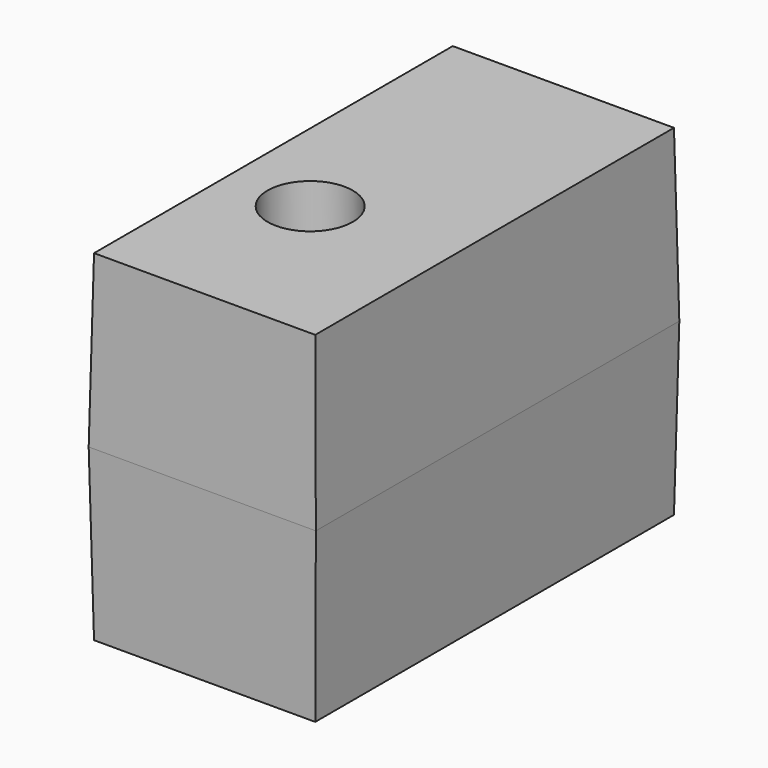
from build123d import *

# Parameters (mm, degrees)
F0_W           = 40
F0_H           = 80
F1_DEPTH       = 30
F1_TAPER       = 1
F3_D           = 9
F3_CBORE_D     = 15
F3_CBORE_DEPTH = 10


with BuildPart() as f1:
    # F0 (on Top) → F1 (new body, symmetric)
    with BuildSketch(Plane.XY):
        with Locations((0, -2.7505960315)):
            Rectangle(F0_W, F0_H)
    extrude(amount=F1_DEPTH, both=True, taper=F1_TAPER)

    # F3 (through all)
    with Locations(Plane.XY.offset(30)):
        with Locations((-5, -12.7505960315)):
            CounterBoreHole(F3_D / 2, F3_CBORE_D / 2, F3_CBORE_DEPTH)


solid = f1.part
